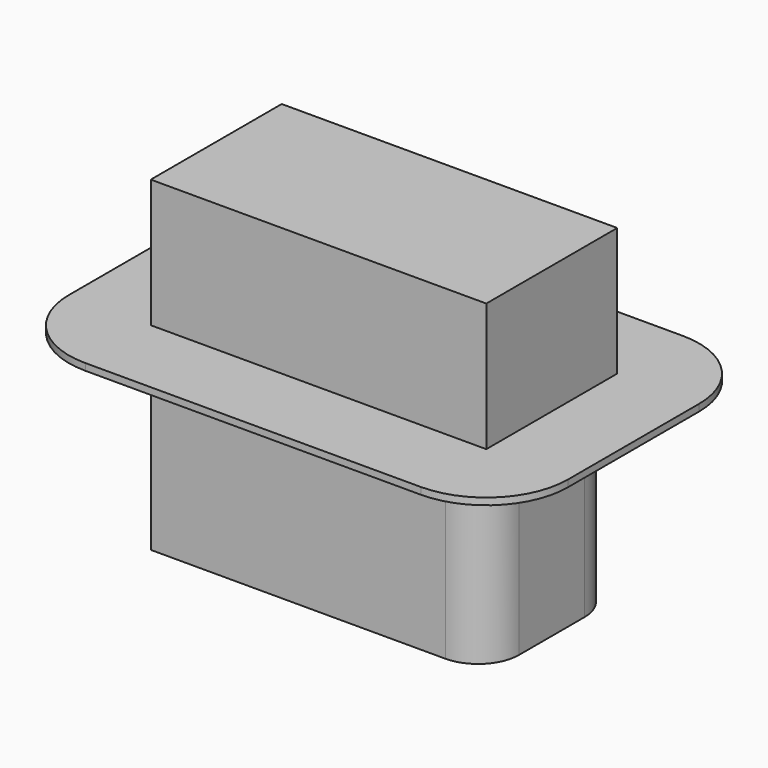
from build123d import *

# Parameters (mm, degrees)
F0_W     = 1230
F0_H     = 600
F1_DEPTH = 470
F2_W     = 1230
F2_H     = 600
F3_DEPTH = 25
F5_DEPTH = 700
F2_W_2   = 300
F6_DEPTH = 150


with BuildPart() as f1:
    # F0 (on Top) → F1 (new body)
    with BuildSketch(Plane.XY):
        Rectangle(F0_W, F0_H)
    extrude(amount=F1_DEPTH)


with BuildPart() as f3:
    # F2 (on face) → F3 (new body)
    with BuildSketch(Plane(origin=(0, 0, 0), x_dir=(1, 0, 0), z_dir=(0, 0, -1))):
        with BuildLine():
            Line((615, 600), (-615, 600))
            ThreePointArc((-615, 600), (-827.132034356, 512.132034356), (-915, 300))
            Line((-915, 300), (-615, 300))
            Line((-615, 300), (615, 300))
            Line((615, 300), (615, -300))
            Line((615, -300), (-615, -300))
            Line((-615, -300), (-915, -300))
            ThreePointArc((-915, -300), (-827.132034356, -512.132034356), (-615, -600))
            Line((-615, -600), (615, -600))
            ThreePointArc((615, -600), (827.132034356, -512.132034356), (915, -300))
            Line((915, -300), (915, 300))
            ThreePointArc((915, 300), (827.132034356, 512.132034356), (615, 600))
        make_face()
        Rectangle(F2_W, F2_H)
    extrude(amount=F3_DEPTH)

    # F4 (on face) → F5 (join)
    with BuildSketch(Plane(origin=(0, 0, -25), x_dir=(1, 0, 0), z_dir=(0, 0, -1))):
        with BuildLine():
            Line((-615, -300), (-465, -300))
            Line((-465, -300), (465, -300))
            ThreePointArc((465, -300), (571.066017178, -256.066017178), (615, -150))
            Line((615, -150), (615, 150))
            ThreePointArc((615, 150), (571.066017178, 256.066017178), (465, 300))
            Line((465, 300), (-465, 300))
            Line((-465, 300), (-615, 300))
            Line((-615, 300), (-615, 150))
            Line((-615, 150), (-615, -150))
            Line((-615, -150), (-615, -300))
        make_face()
    extrude(amount=F5_DEPTH)

    # F2 (on face) → F6 (join)
    with BuildSketch(Plane(origin=(0, 0, 0), x_dir=(1, 0, 0), z_dir=(0, 0, -1))):
        with Locations((-765, 0)):
            Rectangle(F2_W_2, F2_H)
    extrude(amount=F6_DEPTH)


solid = Compound([f1.part, f3.part])
